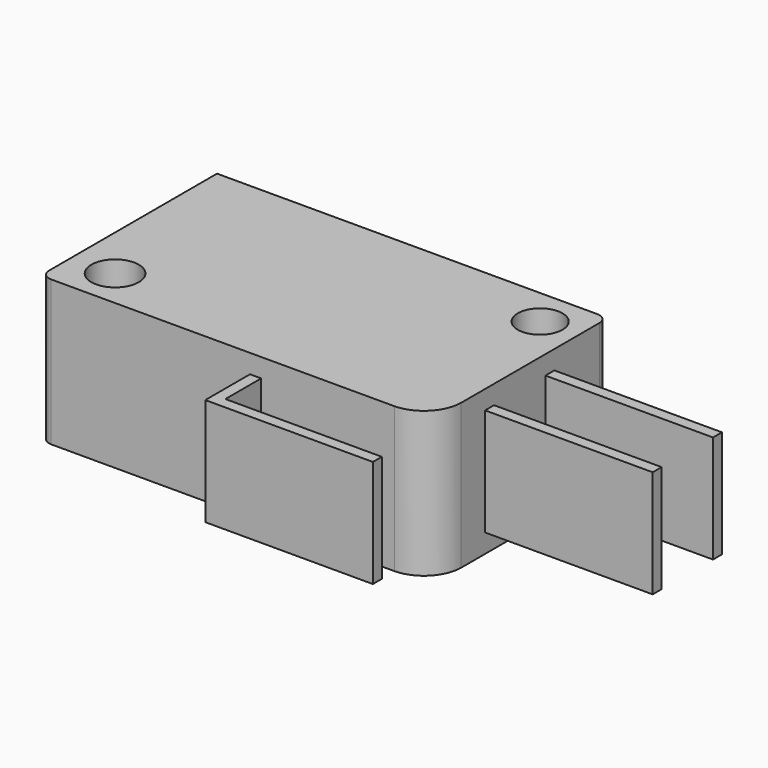
from build123d import *

# Parameters (mm, degrees)
F0_R        = 1.7
F0_R_2      = 1.6
F1_DEPTH    = 10.4
F2_W        = 12.7
F2_H        = 2.7
F2_W_2      = 4
F2_H_2      = 1.35
F3_DEPTH    = 28
F4_W        = 12
F4_H        = 1.35
F5_DEPTH    = 6.2
F6_T1_DEPTH = 23.9048285752
F7_R        = 0.762


# Not quite as in the source:
# - a fillet or chamfer that OpenCascade refuses, or shapes differently, is made with other operations: its cross-section is extruded or revolved along the edge and cut away or added
# - a feature names something its author has since deleted; it is built from what else it names


with BuildPart() as f1:
    # F0 (on Top) → F1 (new body)
    with BuildSketch(Plane.XY):
        with BuildLine():
            Line((3.3782, 0), (0, 0))
            Line((0, 0), (0, -15.8))
            Line((0, -15.8), (15, -15.8))
            Line((15, -15.8), (15, -19.8))
            Line((15, -19.8), (27, -19.8))
            Line((27, -19.8), (27, -19))
            Line((27, -19), (15.8, -19))
            Line((15.8, -19), (15.8, -15.8))
            Line((15.8, -15.8), (28, -15.8))
            Line((28, -15.8), (28, -11))
            Line((28, -11), (40, -11))
            Line((40, -11), (40, -10.2))
            Line((40, -10.2), (28, -10.2))
            Line((28, -10.2), (28, -5.6))
            Line((28, -5.6), (40, -5.6))
            Line((40, -5.6), (40, -4.8))
            Line((40, -4.8), (28, -4.8))
            Line((28, -4.8), (28, 0))
            Line((28, 0), (6.1722, 0))
            Line((6.1722, 0), (6.1722, 1.345))
            ThreePointArc((6.1722, 1.345), (4.7752, 2.742), (3.3782, 1.345))
            Line((3.3782, 1.345), (3.3782, 0))
        make_face()
        with Locations((3.1, -13)):
            Circle(F0_R, mode=Mode.SUBTRACT)
        with Locations((25.3, -2.7)):
            Circle(F0_R_2, mode=Mode.SUBTRACT)
    extrude(amount=F1_DEPTH)

    # F2 (on face) → F3 (cut, through all)
    with BuildSketch(Plane(origin=(0, 0, 0), x_dir=(0, -1, 0), z_dir=(-1, 0, 0))):
        with Locations((-6.35, 9.05)):
            Rectangle(F2_W, F2_H)
        with Locations((-6.35, 1.35)):
            Rectangle(F2_W, F2_H)
        with Locations((17.8, 9.725)):
            Rectangle(F2_W_2, F2_H_2)
        with Locations((17.8, 0.675)):
            Rectangle(F2_W_2, F2_H_2)
    extrude(amount=-F3_DEPTH, mode=Mode.SUBTRACT)

    # F4 (on face) → F5 (cut, through all)
    with BuildSketch(Plane(origin=(0, -4.8, 0), x_dir=(-1, 0, 0), z_dir=(0, 1, 0))):
        with Locations((-34, 9.725)):
            Rectangle(F4_W, F4_H)
        with Locations((-34, 0.675)):
            Rectangle(F4_W, F4_H)
    extrude(amount=-F5_DEPTH, mode=Mode.SUBTRACT)

    # F6: fillet of radius 2.7 on 2 edges, made by hand

    # F6_s2 → F6_t1 (cut)
    with BuildSketch(Plane.XY.offset(-6.7524142876)):
        with BuildLine():
            ThreePointArc((25.2990343146, -15.8004), (27.2091883092, -15.0091883092), (28.0004, -13.0990343146))
            Line((28.0004, -13.0990343146), (28.2705365685, -13.0990343146))
            ThreePointArc((28.2705365685, -13.0990343146), (28.2701365685, -14.4495171573), (28.2701365685, -15.8))
            Line((28.2701365685, -15.8), (28, -16.0701365685))
            ThreePointArc((28, -16.0701365685), (26.6495171573, -16.0701365685), (25.2990343146, -16.0705365685))
            Line((25.2990343146, -16.0705365685), (25.2990343146, -15.8004))
        make_face()
    extrude(amount=F6_T1_DEPTH, mode=Mode.SUBTRACT)

    # F7
    f7_edges = [f1.edges().sort_by_distance(p)[0] for p in [
        (28, 0, 5.2),
        (0, -15.8, 5.2),
    ]]
    fillet(f7_edges, radius=F7_R)


solid = f1.part
